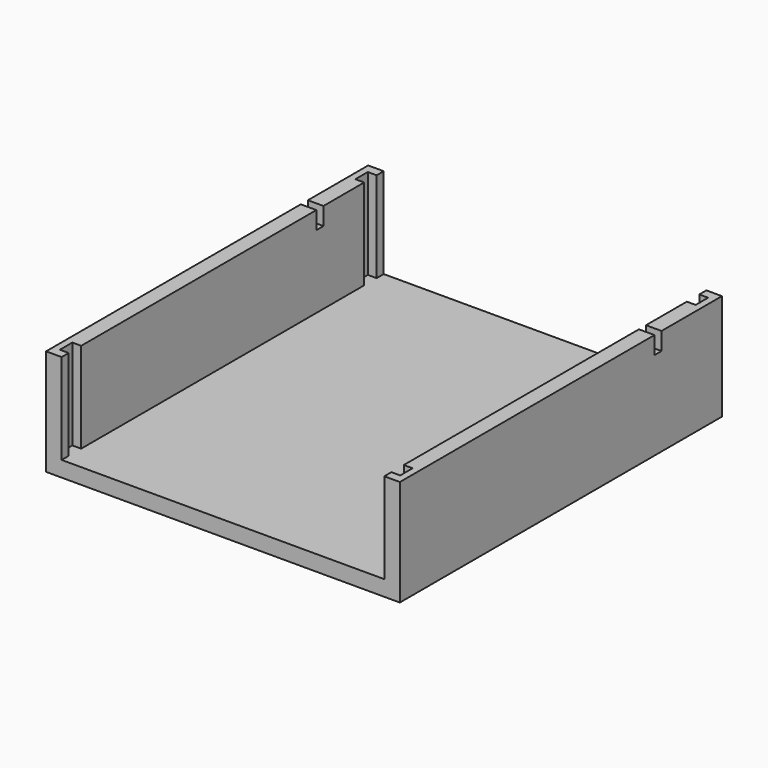
from build123d import *

# Parameters (mm, degrees)
F0_W      = 63.5
F0_H      = 72.263
F1_DEPTH  = 2.794
F2_W      = 2.794
F2_H      = 72.263
F3_DEPTH  = 16.256
F4_W      = 1.5875
F4_H      = 2.794
F5_DEPTH  = 16.256
F6_W      = 1.5875
F6_H      = 2.794
F7_DEPTH  = 16.256
F8_W      = 1.5875
F8_H      = 3.175
F9_DEPTH  = 2.794
F10_W     = 1.5875
F10_H     = 3.174931046
F11_DEPTH = 2.794


# Not quite as in the source:
# - a feature names something its author has since deleted; it is built from what else it names


with BuildPart() as f1:
    # F0 (on Top) → F1 (new body)
    with BuildSketch(Plane.XY):
        Rectangle(F0_W, F0_H)
    extrude(amount=-F1_DEPTH)

    # F2 (on face) → F3 (join)
    with BuildSketch(Plane.XY):
        with Locations((-30.353, 0)):
            Rectangle(F2_W, F2_H)
        with Locations((30.353, 0)):
            Rectangle(F2_W, F2_H)
    extrude(amount=F3_DEPTH)

    # F4 (on face) → F5 (cut, through all)
    with BuildSketch(Plane.XY.offset(16.256)):
        with Locations((-29.74975, 33.147)):
            Rectangle(F4_W, F4_H)
        with Locations((-29.74975, -33.147)):
            Rectangle(F4_W, F4_H)
    extrude(amount=-F5_DEPTH, mode=Mode.SUBTRACT)

    # F6 (on face) → F7 (cut, through all)
    with BuildSketch(Plane.XY.offset(16.256)):
        with Locations((29.74975, 33.147)):
            Rectangle(F6_W, F6_H)
        with Locations((29.74975, -33.147)):
            Rectangle(F6_W, F6_H)
    extrude(amount=-F7_DEPTH, mode=Mode.SUBTRACT)

    # F8 (on face) → F9 (cut, through all)
    with BuildSketch(Plane.YZ.offset(-28.956)):
        with Locations((21.81225, 14.6685)):
            Rectangle(F8_W, F8_H)
    extrude(amount=-F9_DEPTH, mode=Mode.SUBTRACT)

    # F10 (on face) → F11 (cut, through all)
    with BuildSketch(Plane(origin=(28.956, 0, 0), x_dir=(0, -1, 0), z_dir=(-1, 0, 0))):
        with Locations((-21.7913250594, 14.668534477)):
            Rectangle(F10_W, F10_H)
    extrude(amount=-F11_DEPTH, mode=Mode.SUBTRACT)


solid = f1.part
